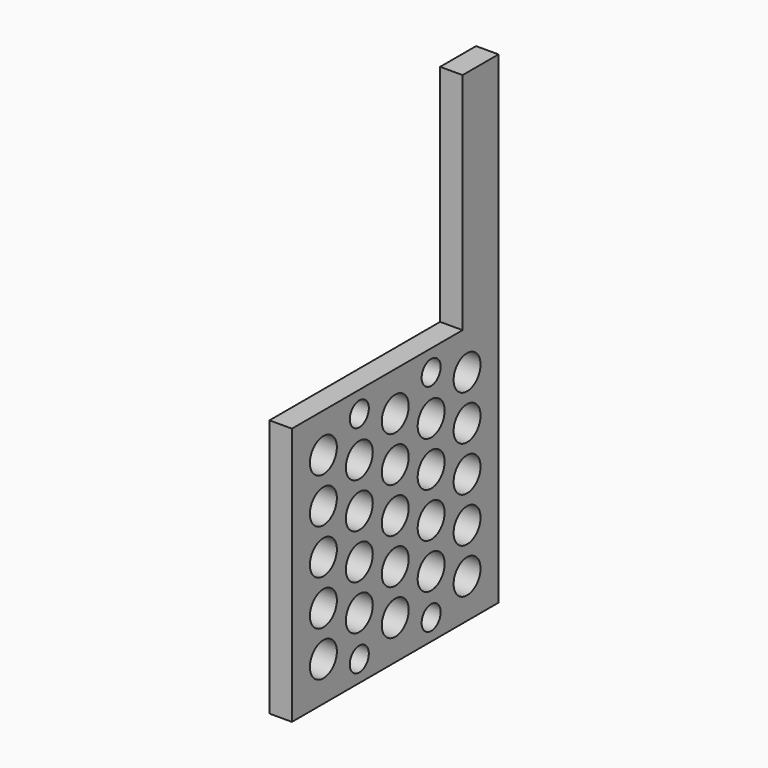
from build123d import *

# Parameters (mm, degrees)
F0_R     = 0.75
F0_R_2   = 0.53
F1_DEPTH = 1


# Not quite as in the source:
# - a feature names something its author has since deleted; it is built from what else it names


with BuildPart() as f1:
    # F0 (on Right) → F1 (new body)
    with BuildSketch(Plane.YZ):
        Polygon((8.384144865, 0), (0, 0), (0, -11.5), (11.5, -11.5), (11.5, 0), (11.2427603453, 0), (10.384144865, 0), (9.499944865, 0), align=None)
        with Locations((1.7500000088, -9.75)):
            Circle(F0_R, mode=Mode.SUBTRACT)
        with Locations((1.75, -7.75)):
            Circle(F0_R, mode=Mode.SUBTRACT)
        with Locations((3.7499851588, -10.5567658602)):
            Circle(F0_R_2, mode=Mode.SUBTRACT)
        with Locations((5.7499653617, -9.750009894)):
            Circle(F0_R, mode=Mode.SUBTRACT)
        with Locations((3.7499885936, -8.7499999912)):
            Circle(F0_R, mode=Mode.SUBTRACT)
        with Locations((3.7499923957, -6.75)):
            Circle(F0_R, mode=Mode.SUBTRACT)
        with Locations((5.7499752647, -7.7500098941)):
            Circle(F0_R, mode=Mode.SUBTRACT)
        with Locations((1.75, -5.75)):
            Circle(F0_R, mode=Mode.SUBTRACT)
        with Locations((1.75, -3.75)):
            Circle(F0_R, mode=Mode.SUBTRACT)
        with Locations((1.75, -1.75)):
            Circle(F0_R, mode=Mode.SUBTRACT)
        with Locations((3.7499961979, -4.75)):
            Circle(F0_R, mode=Mode.SUBTRACT)
        with Locations((5.7499851588, -5.7500098941)):
            Circle(F0_R, mode=Mode.SUBTRACT)
        with Locations((5.7499950529, -3.7500098941)):
            Circle(F0_R, mode=Mode.SUBTRACT)
        with Locations((3.75, -2.75)):
            Circle(F0_R, mode=Mode.SUBTRACT)
        with Locations((3.75, -0.94325)):
            Circle(F0_R_2, mode=Mode.SUBTRACT)
        with Locations((7.749955461, -10.5567658602)):
            Circle(F0_R_2, mode=Mode.SUBTRACT)
        with Locations((7.7499520262, -8.7500197836)):
            Circle(F0_R, mode=Mode.SUBTRACT)
        with Locations((7.7499680167, -6.7500197925)):
            Circle(F0_R, mode=Mode.SUBTRACT)
        with Locations((9.7499307145, -9.750039585)):
            Circle(F0_R, mode=Mode.SUBTRACT)
        with Locations((9.749950516, -7.7500395851)):
            Circle(F0_R, mode=Mode.SUBTRACT)
        with Locations((7.7499840072, -4.7500197926)):
            Circle(F0_R, mode=Mode.SUBTRACT)
        with Locations((5.750004947, -1.7500098941)):
            Circle(F0_R, mode=Mode.SUBTRACT)
        with Locations((7.7499999977, -2.7500197927)):
            Circle(F0_R, mode=Mode.SUBTRACT)
        with Locations((7.7499999977, -0.9432697927)):
            Circle(F0_R_2, mode=Mode.SUBTRACT)
        with Locations((9.7499703087, -5.7500395852)):
            Circle(F0_R, mode=Mode.SUBTRACT)
        with Locations((9.7499901013, -3.7500395853)):
            Circle(F0_R, mode=Mode.SUBTRACT)
        with Locations((9.750009894, -1.7500395854)):
            Circle(F0_R, mode=Mode.SUBTRACT)
        Polygon((9.499944865, 10), (9.499944865, 0), (10.384144865, 0), (11.2427603453, 0), (11.5, 0), (11.5, 10), (10.384144865, 10), align=None)
    extrude(amount=F1_DEPTH)


solid = f1.part
